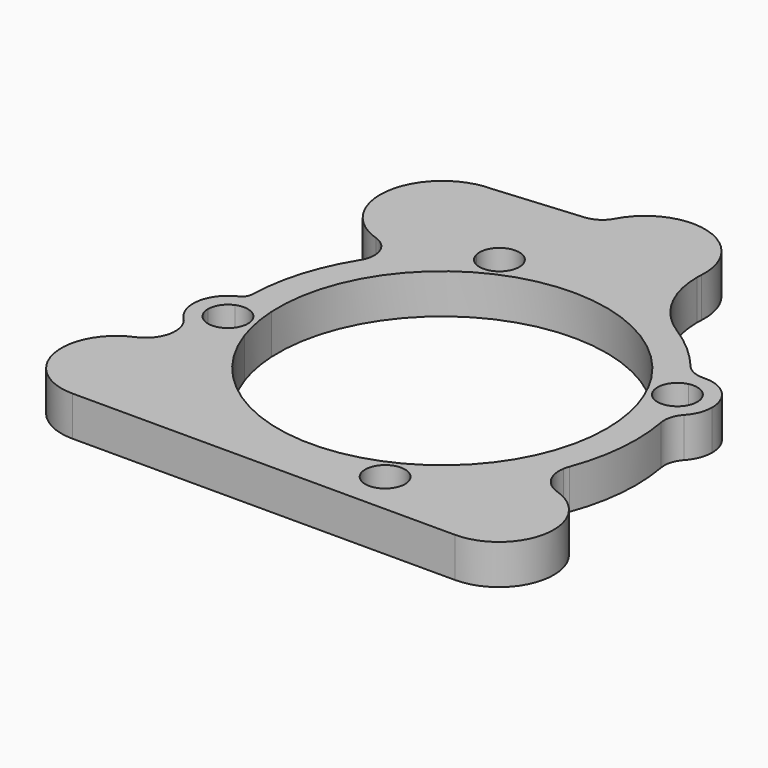
from build123d import *

# Parameters (mm, degrees)
F0_R     = 6.35
F1_DEPTH = 12.7
F2_R     = 7.9375


with BuildPart() as f1:
    # F0 (on Top) → F1 (new body)
    with BuildSketch(Plane.XY):
        with BuildLine():
            ThreePointArc((50.0804162666, 15.375371957), (51.8075185828, 7.7737490661), (52.3875, 0))
            ThreePointArc((52.3875, 0), (8.6161289731, -51.6740987127), (-49.5533247299, -16.9975929021))
            ThreePointArc((-49.5533247299, -16.9975929021), (-51.4249940729, -9.9960062453), (-52.312453003, -2.8031084642))
            ThreePointArc((-52.312453003, -2.8031084642), (-56.8688591942, -0.6489004527), (-61.9082087133, -0.7289376965))
            ThreePointArc((-61.9082087133, -0.7289376965), (-61.8302354833, -3.1905542348), (-61.6544213285, -5.6471220008))
            ThreePointArc((-61.6544213285, -5.6471220008), (-55.692265244, -6.2283994183), (-52.8666598415, -11.5105526461))
            ThreePointArc((-52.8666598415, -11.5105526461), (-59.2166598415, -17.8605526461), (-65.5666598415, -11.5105526461))
            Line((-65.5666598415, -11.5105526461), (-70.3291598415, -11.5105526461))
            ThreePointArc((-70.3291598415, -11.5105526461), (-69.508132002, -15.702599523), (-67.166368927, -19.2752021362))
            ThreePointArc((-67.166368927, -19.2752021362), (-65.1591434342, -22.3374329476), (-64.4554052861, -25.9306159849))
            ThreePointArc((-64.4554052861, -25.9306159849), (-66.044465468, -31.1981091461), (-70.2814387145, -34.7080456373))
            ThreePointArc((-70.2814387145, -34.7080456373), (-80.6164344901, -54.2592739984), (-63.5, -68.2625))
            Line((-63.5, -68.2625), (0, -68.2625))
            Line((0, -68.2625), (58.7375, -68.2625))
            ThreePointArc((58.7375, -68.2625), (75.9947089073, -53.4697653418), (64.0142585669, -34.153837521))
            ThreePointArc((64.0142585669, -34.153837521), (58.7813342607, -30.0675851979), (57.4893859738, -23.5551490588))
            ThreePointArc((57.4893859738, -23.5551490588), (57.686142675, -22.631002937), (57.9734917775, -21.7308975281))
            ThreePointArc((57.9734917775, -21.7308975281), (61.831190131, -3.1719998798), (59.8929243466, 15.6842363367))
            ThreePointArc((59.8929243466, 15.6842363367), (55.0226278067, 14.3874475529), (50.0804162666, 15.375371957))
        make_face()
        with Locations((25.4944466395, -54.673017253)):
            Circle(F0_R, mode=Mode.SUBTRACT)
        with BuildLine():
            ThreePointArc((43.9692893127, 28.4807260018), (47.4791991934, 22.1399141869), (50.0804162666, 15.375371957))
            ThreePointArc((50.0804162666, 15.375371957), (55.0226278067, 14.3874475529), (59.8929243466, 15.6842363367))
            ThreePointArc((59.8929243466, 15.6842363367), (59.2217483156, 18.053868912), (58.456859062, 20.394932823))
            ThreePointArc((58.456859062, 20.394932823), (48.9179628053, 22.8108206775), (53.1987696631, 31.6709419276))
            ThreePointArc((53.1987696631, 31.6709419276), (51.8970719981, 33.7616879655), (50.5132517682, 35.7990090932))
            ThreePointArc((50.5132517682, 35.7990090932), (46.3892876551, 32.9017052551), (43.9692893127, 28.4807260018))
        make_face()
        with BuildLine():
            ThreePointArc((-52.312453003, -2.8031084642), (-16.1886277928, 49.8234732474), (43.9692893127, 28.4807260018))
            ThreePointArc((43.9692893127, 28.4807260018), (46.3892876551, 32.9017052551), (50.5132517682, 35.7990090932))
            ThreePointArc((50.5132517682, 35.7990090932), (52.310310906, 36.3528661823), (54.1750282482, 36.5957827393))
            ThreePointArc((54.1750282482, 36.5957827393), (50.6015982243, 37.2692654479), (47.7034897917, 39.4656143744))
            ThreePointArc((47.7034897917, 39.4656143744), (40.8771414604, 46.4996447543), (33.0262233797, 52.3681795132))
            ThreePointArc((33.0262233797, 52.3681795132), (17.1888443577, 59.4785783783), (-4.35e-08, 61.9125))
            ThreePointArc((-4.35e-08, 61.9125), (-10.3428083822, 61.0424767766), (-20.394932823, 58.456859062))
            ThreePointArc((-20.394932823, 58.456859062), (-19.4651675477, 56.6655768212), (-19.1444466395, 54.673017253))
            ThreePointArc((-19.1444466395, 54.673017253), (-24.7522354429, 48.3665426007), (-31.6709419276, 53.1987696631))
            ThreePointArc((-31.6709419276, 53.1987696631), (-43.3001474916, 44.252173771), (-52.4975053225, 32.8202618997))
            ThreePointArc((-52.4975053225, 32.8202618997), (-59.2888527637, 17.8322627339), (-61.8922171982, 1.5846471339))
            ThreePointArc((-61.8922171982, 1.5846471339), (-62.4517909232, -0.1996749025), (-63.8695481256, -1.4190568766))
            ThreePointArc((-63.8695481256, -1.4190568766), (-68.5759567517, -5.5196247049), (-70.3291598415, -11.5105526461))
            Line((-70.3291598415, -11.5105526461), (-65.5666598415, -11.5105526461))
            ThreePointArc((-65.5666598415, -11.5105526461), (-64.4988130692, -7.9861580486), (-61.6544213285, -5.6471220008))
            ThreePointArc((-61.6544213285, -5.6471220008), (-61.8302354833, -3.1905542348), (-61.9082087133, -0.7289376965))
            ThreePointArc((-61.9082087133, -0.7289376965), (-56.8688591942, -0.6489004527), (-52.312453003, -2.8031084642))
        make_face()
        with BuildLine():
            ThreePointArc((58.456859062, 20.394932823), (59.2217483156, 18.053868912), (59.8929243466, 15.6842363367))
            ThreePointArc((59.8929243466, 15.6842363367), (64.1991359229, 19.7724959812), (65.785517253, 25.4944466395))
            ThreePointArc((65.785517253, 25.4944466395), (62.3526576558, 33.526306918), (54.1750282482, 36.5957827393))
            ThreePointArc((54.1750282482, 36.5957827393), (52.310310906, 36.3528661823), (50.5132517682, 35.7990090932))
            ThreePointArc((50.5132517682, 35.7990090932), (51.8970719981, 33.7616879655), (53.1987696631, 31.6709419276))
            ThreePointArc((53.1987696631, 31.6709419276), (58.6075456748, 30.4786202017), (61.023017253, 25.4944466395))
            ThreePointArc((61.023017253, 25.4944466395), (60.3453137671, 22.6400548906), (58.456859062, 20.394932823))
        make_face()
        with BuildLine():
            ThreePointArc((-4.35e-08, 61.9125), (17.1888443577, 59.4785783783), (33.0262233797, 52.3681795132))
            ThreePointArc((33.0262233797, 52.3681795132), (22.7049210277, 63.3125798927), (18.9534219493, 77.8808823529))
            ThreePointArc((18.9534219493, 77.8808823529), (18.9682238309, 78.8257127153), (19.0126149481, 79.7696157495))
            ThreePointArc((19.0126149481, 79.7696157495), (13.041818397, 67.0767708906), (-4.35e-08, 61.9125))
        make_face()
        with BuildLine():
            ThreePointArc((-20.394932823, 58.456859062), (-10.3428083822, 61.0424767766), (-4.35e-08, 61.9125))
            ThreePointArc((-4.35e-08, 61.9125), (-3.8885649879, 62.3135975568), (-7.6133825433, 63.5))
            Line((-7.6133825433, 63.5), (-50.8, 63.5))
            Line((-50.8, 63.5), (-70.64375, 63.5))
            ThreePointArc((-70.64375, 63.5), (-66.8192563388, 51.788559422), (-56.8199676592, 44.5914198459))
            ThreePointArc((-56.8199676592, 44.5914198459), (-51.7769282768, 39.7640636512), (-52.4975053225, 32.8202618997))
            ThreePointArc((-52.4975053225, 32.8202618997), (-43.3001474916, 44.252173771), (-31.6709419276, 53.1987696631))
            ThreePointArc((-31.6709419276, 53.1987696631), (-28.1780726016, 60.4280717007), (-20.394932823, 58.456859062))
        make_face()
        with BuildLine():
            ThreePointArc((-7.6133825433, 63.5), (-3.8885649879, 62.3135975568), (-4.35e-08, 61.9125))
            ThreePointArc((-4.35e-08, 61.9125), (13.041818397, 67.0767708906), (19.0126149481, 79.7696157495))
            ThreePointArc((19.0126149481, 79.7696157495), (5.2010600776, 99.2887509551), (-16.8048050509, 89.934736466))
            ThreePointArc((-16.8048050509, 89.934736466), (-19.4314787596, 87.050449272), (-23.1150084474, 85.7658729107))
            Line((-23.1150084474, 85.7658729107), (-50.8, 83.34375))
            ThreePointArc((-50.8, 83.34375), (-64.8316501892, 77.5316501892), (-70.64375, 63.5))
            Line((-70.64375, 63.5), (-50.8, 63.5))
            Line((-50.8, 63.5), (-7.6133825433, 63.5))
        make_face()
    extrude(amount=F1_DEPTH)

    # F2
    f2_edges = [f1.edges().sort_by_distance(p)[0] for p in [
        (59.892924, 15.684236, 6.35),
    ]]
    fillet(f2_edges, radius=F2_R)


solid = f1.part
